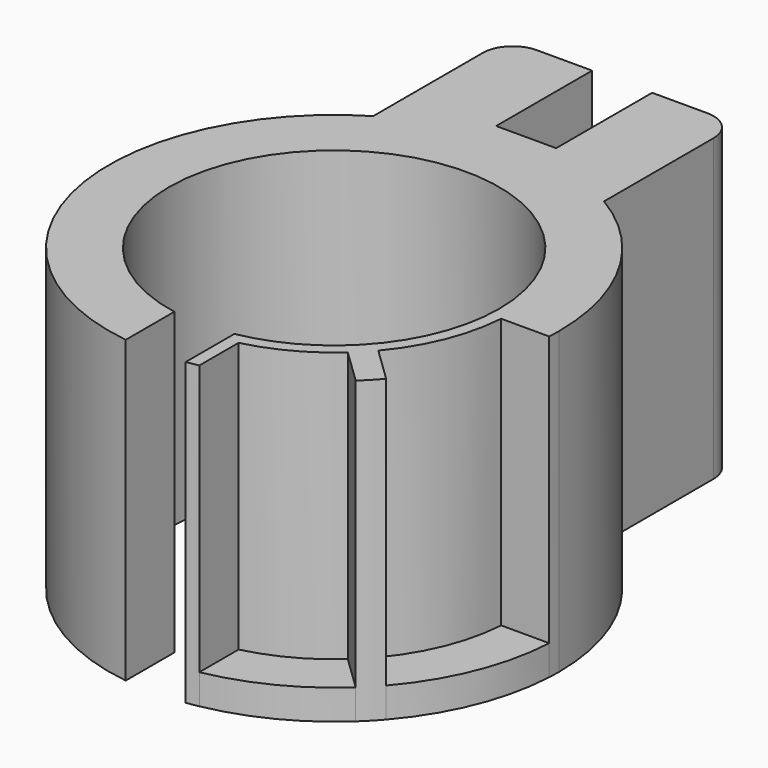
from build123d import *

# Parameters (mm, degrees)
F1_DEPTH = 50
F2_DEPTH = 5


# Not quite as in the source:
# - a feature of the source that left no trace in its solid (it failed there, or was rolled back) is left out


with BuildPart() as f1:
    # F0 (on Top) → F1 (new body)
    with BuildSketch(Plane.XY):
        with BuildLine():
            Line((-19.2333690145, -5), (-19.2333690145, -27.8079588042))
            ThreePointArc((-19.2333690145, -27.8079588042), (-36.7344496958, -67.5385811362), (-5, -97.1651718683))
            Line((-5, -97.1651718683), (-5, -87.041634566))
            ThreePointArc((-5, -87.041634566), (-17.5890590993, -38.8605818434), (27.5, -60))
            ThreePointArc((27.5, -60), (25.4982682633, -70.2999182314), (19.7844861402, -79.1003693203))
            ThreePointArc((19.7844861402, -79.1003693203), (13.0128248945, -84.2263573049), (5, -87.041634566))
            Line((5, -87.041634566), (5, -97.1651718683))
            ThreePointArc((5, -97.1651718683), (6.0021906226, -97.0165328972), (7, -96.8408740396))
            Line((7, -96.8408740396), (7, -88.6574597618))
            ThreePointArc((7, -88.6574597618), (13.8146262679, -86.0654196413), (19.7854086015, -81.8812158362))
            Line((19.7854086015, -81.8812158362), (25.5513297312, -87.4477603634))
            ThreePointArc((25.5513297312, -87.4477603634), (26.9788447366, -86.045958164), (28.3295652687, -84.5700169249))
            Line((28.3295652687, -84.5700169249), (22.563644139, -79.0034723976))
            ThreePointArc((22.563644139, -79.0034723976), (27.3526877734, -71.0490031936), (29.4321253055, -62))
            Line((29.4321253055, -62), (37.4466286867, -62))
            ThreePointArc((37.4466286867, -62), (37.4866547971, -61.0003559988), (37.5, -60))
            ThreePointArc((37.5, -60), (32.6151907709, -41.4932625517), (19.2333690145, -27.8079588042))
            Line((19.2333690145, -27.8079588042), (19.2333690145, -5))
            ThreePointArc((19.2333690145, -5), (17.7689029204, -1.4644660941), (14.2333690145, 0))
            Line((14.2333690145, 0), (5, 0))
            Line((5, 0), (5, -20))
            Line((5, -20), (0, -20))
            Line((0, -20), (-5, -20))
            Line((-5, -20), (-5, 0))
            Line((-5, 0), (-14.2333690145, 0))
            ThreePointArc((-14.2333690145, 0), (-17.7689029204, -1.4644660941), (-19.2333690145, -5))
        make_face()
    extrude(amount=F1_DEPTH)

    # F0 (on Top) → F2 (join)
    with BuildSketch(Plane.XY):
        with BuildLine():
            Line((7, -88.6574597618), (7, -96.8408740396))
            ThreePointArc((7, -96.8408740396), (16.9397435916, -93.4558677522), (25.5513297312, -87.4477603634))
            Line((25.5513297312, -87.4477603634), (19.7854086015, -81.8812158362))
            ThreePointArc((19.7854086015, -81.8812158362), (13.8146262679, -86.0654196413), (7, -88.6574597618))
        make_face()
        with BuildLine():
            Line((22.563644139, -79.0034723976), (28.3295652687, -84.5700169249))
            ThreePointArc((28.3295652687, -84.5700169249), (34.7703658136, -74.0453430428), (37.4466286867, -62))
            Line((37.4466286867, -62), (29.4321253055, -62))
            ThreePointArc((29.4321253055, -62), (27.3526877734, -71.0490031936), (22.563644139, -79.0034723976))
        make_face()
    extrude(amount=F2_DEPTH)


solid = f1.part
